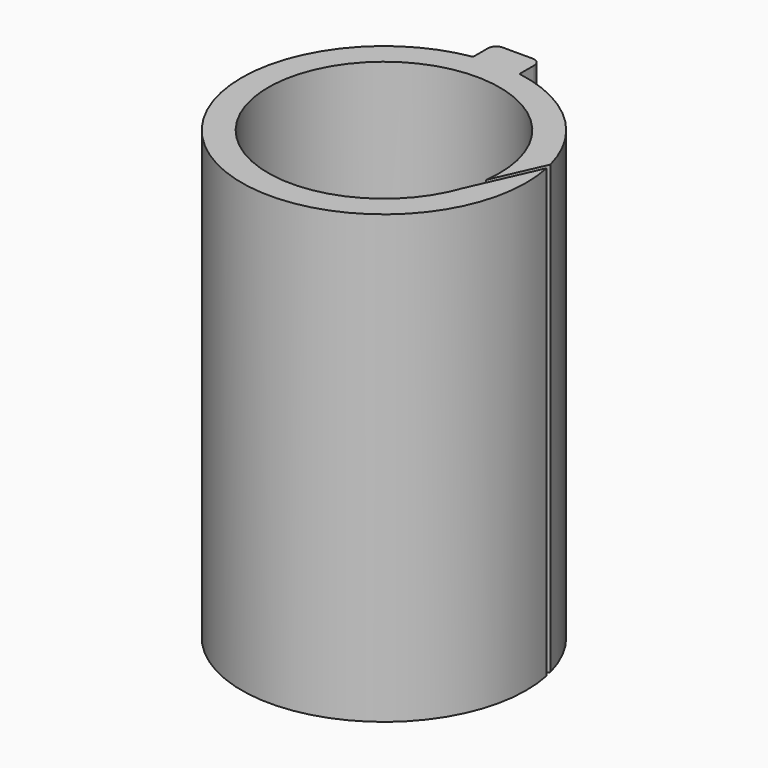
from build123d import *

# Parameters (mm, degrees)
F1_DEPTH = 27
F2_DEPTH = 18
F3_R     = 1.9999
F4_R     = 0.5


# Not quite as in the source:
# - a fillet or chamfer is up to 0.001 mm smaller than in the source, because OpenCascade refuses the exact size


with BuildPart() as f1:
    # F0 (on Top) → F1 (new body)
    with BuildSketch(Plane.XY):
        with BuildLine():
            ThreePointArc((6.6154708154, -2.2881315283), (4.8415745742, -5.0556063576), (2, -6.7082039325))
            ThreePointArc((2, -6.7082039325), (0, -7), (-2, -6.7082039325))
            ThreePointArc((-2, -6.7082039325), (-3.7888849897, 5.8859451692), (6.9342650073, -0.9570625938))
            Line((6.9342650073, -0.9570625938), (8.3233295817, 2.1638356393))
            ThreePointArc((8.3233295817, 2.1638356393), (5.7987889756, 6.3509091015), (1.4, 8.4852813742))
            Line((1.4, 8.4852813742), (1.4, 10.1))
            Line((1.4, 10.1), (-1.4, 10.1))
            Line((-1.4, 10.1), (-1.4, 8.4852813742))
            ThreePointArc((-1.4, 8.4852813742), (-4.8595970429, -7.0953728994), (8.4177416777, 1.7611431082))
            Line((8.4177416777, 1.7611431082), (6.6154708154, -2.2881315283))
        make_face()
    extrude(amount=F1_DEPTH)

    # F0 (on Top) → F2 (join)
    with BuildSketch(Plane.XY):
        with BuildLine():
            ThreePointArc((-2, -6.7082039325), (0, -7), (2, -6.7082039325))
            Line((2, -6.7082039325), (2, -5))
            Line((2, -5), (-2, -5))
            Line((-2, -5), (-2, -6.7082039325))
        make_face()
        with BuildLine():
            ThreePointArc((6.6154708154, -2.2881315283), (4.8415745742, -5.0556063576), (2, -6.7082039325))
            ThreePointArc((2, -6.7082039325), (0, -7), (-2, -6.7082039325))
            ThreePointArc((-2, -6.7082039325), (-3.7888849897, 5.8859451692), (6.9342650073, -0.9570625938))
            Line((6.9342650073, -0.9570625938), (8.3233295817, 2.1638356393))
            ThreePointArc((8.3233295817, 2.1638356393), (5.7987889756, 6.3509091015), (1.4, 8.4852813742))
            Line((1.4, 8.4852813742), (1.4, 10.1))
            Line((1.4, 10.1), (-1.4, 10.1))
            Line((-1.4, 10.1), (-1.4, 8.4852813742))
            ThreePointArc((-1.4, 8.4852813742), (-4.8595970429, -7.0953728994), (8.4177416777, 1.7611431082))
            Line((8.4177416777, 1.7611431082), (6.6154708154, -2.2881315283))
        make_face()
    extrude(amount=F2_DEPTH)

    # F3 (radius 2 in the source; OpenCascade refuses exactly that, so slightly less here)
    f3_edges = [f1.edges().sort_by_distance(p)[0] for p in [
        (2, -5.854102, 18),
        (-2, -5.854102, 18),
        (2, -5.854102, 0),
        (-2, -5.854102, 0),
    ]]
    fillet(f3_edges, radius=F3_R)

    # F4
    f4_edges = [f1.edges().sort_by_distance(p)[0] for p in [
        (2, -5, 9),
        (1.4, 10.1, 13.5),
        (-1.4, 10.1, 13.5),
    ]]
    fillet(f4_edges, radius=F4_R)


solid = f1.part
